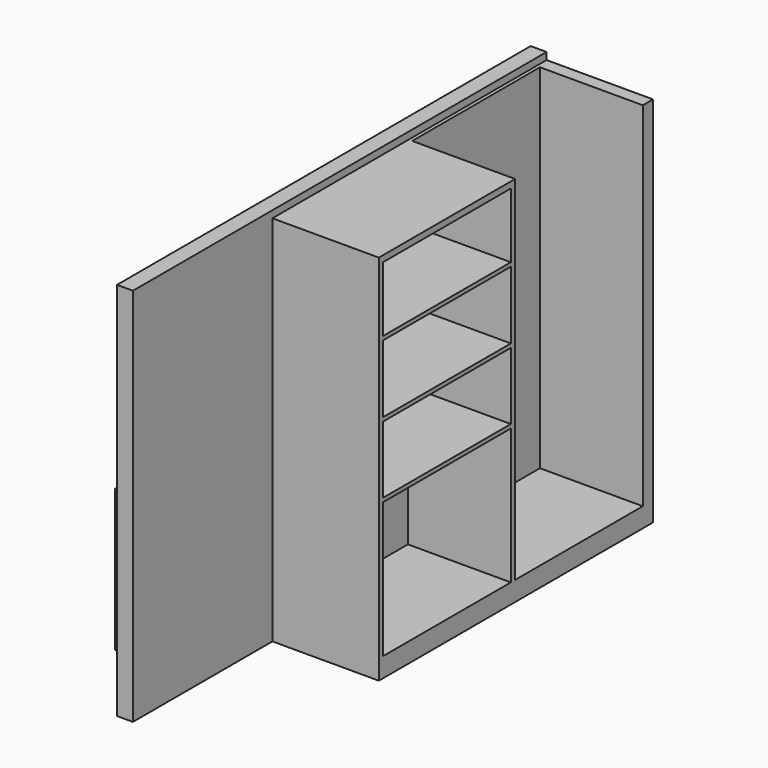
from build123d import *

# Parameters (mm, degrees)
F0_W      = 205
F0_H      = 1140
F0_W_2    = 799
F0_H_2    = 290
F1_DEPTH  = 500
F2_W      = 95
F2_H      = 60
F3_DEPTH  = 100
F4_W      = 2915
F4_H      = 2140
F5_DEPTH  = 90
F6_W      = 1860
F6_H      = 110
F7_DEPTH  = 600
F6_H_2    = 1990
F8_DEPTH  = 20
F9_R      = 5
F10_DEPTH = 760.001
F11_W     = 30
F11_H     = 1990
F12_DEPTH = 580
F13_W     = 1080
F13_H     = 625
F14_DEPTH = 120
F13_W_2   = 1180
F13_H_2   = 800
F15_DEPTH = 400
F16_R     = 10
F17_DEPTH = 110
F18_W     = 900
F18_H     = 35
F18_H_2   = 22
F19_DEPTH = 580


# Not quite as in the source:
# - a feature names something its author has since deleted; it is built from what else it names


with BuildPart() as f1:
    # F0 (on Right) → F1 (new body)
    with BuildSketch(Plane.YZ):
        Polygon((0, -53), (0, 0), (-205, 0), (-899, 0), (-899, -53), (-799, -53), align=None)
        with Locations((-102.5, 570)):
            Rectangle(F0_W, F0_H)
        Polygon((-205, 1140), (0, 1140), (0, 1187), (-265, 1187), (-265, 1140), align=None)
        with Locations((-399.5, -198)):
            Rectangle(F0_W_2, F0_H_2)
    extrude(amount=-F1_DEPTH)

    # F2 (on face) → F3 (cut)
    with BuildSketch(Plane.XZ.offset(205)):
        with Locations((-117.5, 144)):
            Rectangle(F2_W, F2_H)
    extrude(amount=-F3_DEPTH, mode=Mode.SUBTRACT)

    # F4 (on Right) → F5 (join)
    with BuildSketch(Plane.YZ):
        with Locations((-1457.5, 727)):
            Rectangle(F4_W, F4_H)
    extrude(amount=F5_DEPTH)

    # F9 (on face) → F10 (cut, through all)
    with BuildSketch(Plane(origin=(-70, 0, 0), x_dir=(0, -1, 0), z_dir=(-1, 0, 0))):
        with Locations((125, 144)):
            Circle(F9_R)
    extrude(amount=-F10_DEPTH, mode=Mode.SUBTRACT)

    # F16 (on face) → F17 (cut, through all)
    with BuildSketch(Plane(origin=(0, 0, 0), x_dir=(0, -1, 0), z_dir=(-1, 0, 0))):
        with Locations((1385, 1157)):
            Circle(F16_R)
    extrude(amount=-F17_DEPTH, mode=Mode.SUBTRACT)


with BuildPart() as f7:
    # F6 (on face) → F7 (new body)
    with BuildSketch(Plane.YZ.offset(90)):
        Polygon((-72, -343), (0, -343), (0, 1757), (-72, 1757), (-72, -233), align=None)
        with Locations((-1002, -288)):
            Rectangle(F6_W, F6_H)
    extrude(amount=F7_DEPTH)

    # F6 (on face) → F8 (join)
    with BuildSketch(Plane.YZ.offset(90)):
        Polygon((-72, -343), (0, -343), (0, 1757), (-72, 1757), (-72, -233), align=None)
        with Locations((-1002, -288)):
            Rectangle(F6_W, F6_H)
        with Locations((-1002, 762)):
            Rectangle(F6_W, F6_H_2)
    extrude(amount=F8_DEPTH)

    # F11 (on face) → F12 (join, through all)
    with BuildSketch(Plane.YZ.offset(110)):
        with Locations((-987, 762)):
            Rectangle(F11_W, F11_H)
        with Locations((-1917, 762)):
            Rectangle(F11_W, F11_H)
    extrude(amount=F12_DEPTH)

    # F18 (on face) → F19 (join, through all)
    with BuildSketch(Plane.YZ.offset(110)):
        with Locations((-1452, 1739.5)):
            Rectangle(F18_W, F18_H)
        with Locations((-1452, 1345)):
            Rectangle(F18_W, F18_H_2)
        with Locations((-1452, 942)):
            Rectangle(F18_W, F18_H_2)
        with Locations((-1452, 542)):
            Rectangle(F18_W, F18_H_2)
    extrude(amount=F19_DEPTH)


with BuildPart() as f14:
    # F13 (on face) → F14 (new body)
    with BuildSketch(Plane(origin=(0, 0, 0), x_dir=(0, -1, 0), z_dir=(-1, 0, 0))):
        with Locations((1840, 1047)):
            Rectangle(F13_W, F13_H)
    extrude(amount=F14_DEPTH)


with BuildPart() as f15:
    # F13 (on face) → F15 (new body)
    with BuildSketch(Plane(origin=(0, 0, 0), x_dir=(0, -1, 0), z_dir=(-1, 0, 0))):
        with Locations((1839, 57)):
            Rectangle(F13_W_2, F13_H_2)
    extrude(amount=F15_DEPTH)


solid = Compound([f1.part, f7.part, f14.part, f15.part])
